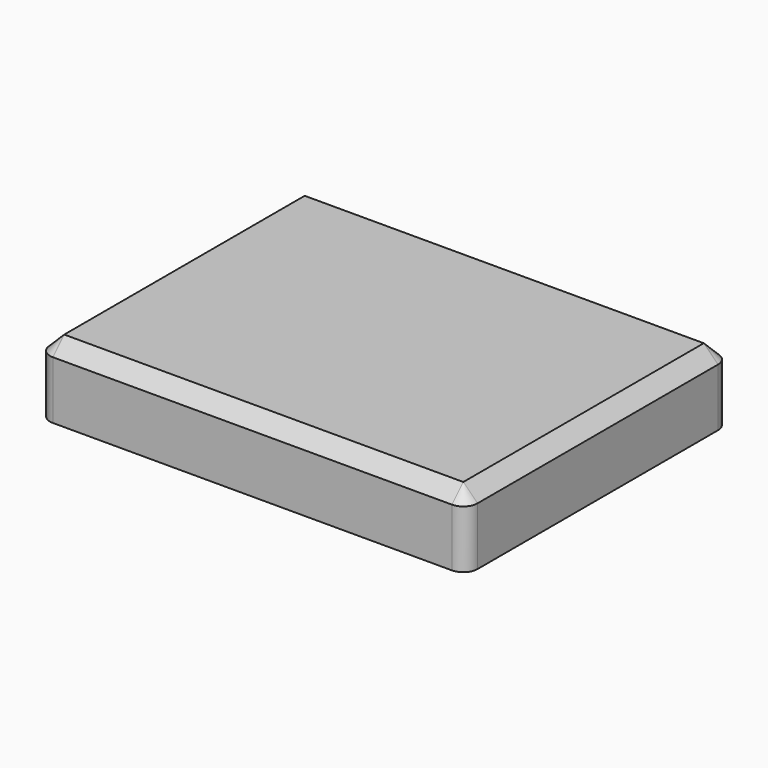
from build123d import *

# Parameters (mm, degrees)
F0_W     = 150.6762728095
F0_H     = 115.9463040531
F1_DEPTH = 25.4
F2_R     = 5
F3_SIZE  = 5
F4_T     = 2.5


# Not quite as in the source:
# - a shell that OpenCascade refuses in one call is made with other operations: the cavity is built on its own and cut out


with BuildPart() as f1:
    # F0 (on Top) → F1 (new body)
    with BuildSketch(Plane.XY):
        with Locations((-0.7436312735, 18.0544536561)):
            Rectangle(F0_W, F0_H)
    extrude(amount=F1_DEPTH)

    # F2
    f2_edges = [f1.edges().sort_by_distance(p)[0] for p in [
        (-76.081768, -39.918698, 12.7),
        (74.594505, -39.918698, 12.7),
        (74.594505, 76.027606, 12.7),
    ]]
    fillet(f2_edges, radius=F2_R)

    # F3
    f3_edges = [f1.edges().sort_by_distance(p)[0] for p in [
        (-76.081768, 20.554454, 25.4),
        (-74.617302, -38.454232, 25.4),
        (-3.243631, 76.027606, 25.4),
        (-0.743631, -39.918698, 25.4),
        (73.130039, 74.56314, 25.4),
        (73.130039, -38.454232, 25.4),
        (74.594505, 18.054454, 25.4),
    ]]
    chamfer(f3_edges, length=F3_SIZE)

    # F4: shell of thickness 2.5, made by hand


with BuildPart() as f4_core1:
    # F4_t2: copy of F1
    add(f1.part)

    # the walls: a layer under each face that stays
    f4_faces = [f4_core1.faces().sort_by_distance(p)[0] for p in [
        (-76.0817676783, 20.5544536561, 10.2),
        (-74.6173015842, -38.4542322764, 10.2),
        (-73.5817676783, 20.5544536561, 22.9),
        (-3.2436312735, 76.0276056826, 10.2),
        (-72.8495346312, -36.6864653234, 22.9),
        (-0.7436312735, -39.9186983705, 10.2),
        (-3.2436312735, 73.5276056826, 22.9),
        (-0.7436312735, 18.0544536561, 25.4),
        (73.1300390372, 74.5631395885, 10.2),
        (73.1300390372, -38.4542322764, 10.2),
        (74.5945051312, 18.0544536561, 10.2),
        (-0.7436312735, -37.4186983705, 22.9),
        (71.3622720842, 72.7953726356, 22.9),
        (72.0945051312, 18.0544536561, 22.9),
        (71.3622720842, -36.6864653234, 22.9),
    ]]
    thicken(f4_faces, amount=-F4_T, mode=Mode.SUBTRACT)


with BuildPart() as f1_1:
    add(f1.part)

    # what is left inside the walls is the cavity
    f4_cavity = [f4_core1.part.solids().sort_by_distance(p)[0] for p in [
        (-0.743631, -0.436597, 0.025),
    ]]
    add(f4_cavity, mode=Mode.SUBTRACT)


solid = f1_1.part
